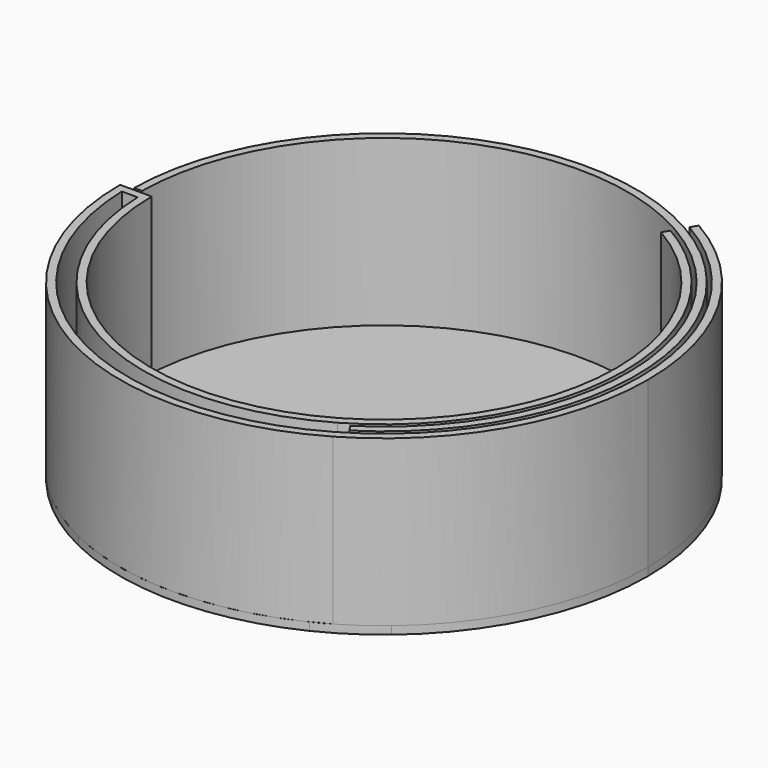
from build123d import *

# Parameters (mm, degrees)
F1_DEPTH = 1.2
F3_DEPTH = 25


with BuildPart() as f1:
    # F0 (on Top) → F1 (new body)
    with BuildSketch(Plane.XY):
        with BuildLine():
            ThreePointArc((25.666348, -30.679612), (36.239853, -16.931422), (40, 0))
            ThreePointArc((40, 0), (-16.931422, 36.239853), (-25.666348, -30.679612))
            ThreePointArc((-25.666348, -30.679612), (-21.736946, -33.578344), (-17.483625, -35.976699))
            ThreePointArc((-17.483625, -35.976699), (0, -40), (17.483625, -35.976699))
            ThreePointArc((17.483625, -35.976699), (21.736946, -33.578344), (25.666348, -30.679612))
        make_face()
    extrude(amount=F1_DEPTH)

    # F2 (on face) → F3 (join)
    with BuildSketch(Plane.XY.offset(1.2)):
        with BuildLine():
            ThreePointArc((20, -34.641016), (34.641016, -20), (40, 0))
            ThreePointArc((40, 0), (34.641016, 20), (20, 34.641016))
            Line((20, 34.641016), (19.4, 33.601786))
            ThreePointArc((19.4, 33.601786), (33.601786, 19.4), (38.8, 0))
            ThreePointArc((38.8, 0), (33.601786, -19.4), (19.4, -33.601786))
            Line((19.4, -33.601786), (20, -34.641016))
        make_face()
        with BuildLine():
            ThreePointArc((-40, 0), (-20, -34.641016), (20, -34.641016))
            Line((20, -34.641016), (19.4, -33.601786))
            ThreePointArc((19.4, -33.601786), (-18.878002, -33.897803), (-38.781439, -1.2))
            ThreePointArc((-38.781439, -1.2), (-38.795359, -0.600072), (-38.8, 0))
            Line((-38.8, 0), (-40, 0))
        make_face()
        with BuildLine():
            Line((18.5, 32.04294), (19.1, 33.08217))
            ThreePointArc((19.1, 33.08217), (-18.920896, 33.184932), (-38.197768, 0.412973))
            Line((-38.197768, 0.412973), (-36.997838, 0.4))
            ThreePointArc((-36.997838, 0.4), (-18.326522, 32.142473), (18.5, 32.04294))
        make_face()
        with BuildLine():
            ThreePointArc((20.512714, -32.225279), (38.191066, 0.826139), (19.1, 33.08217))
            Line((19.1, 33.08217), (18.5, 32.04294))
            ThreePointArc((18.5, 32.04294), (36.991346, 0.800187), (19.868335, -31.212966))
            Line((19.868335, -31.212966), (20.512714, -32.225279))
        make_face()
        with BuildLine():
            Line((17.6, -30.484094), (18.2, -31.523325))
            ThreePointArc((18.2, -31.523325), (31.523325, -18.2), (36.4, 0))
            ThreePointArc((36.4, 0), (31.523325, 18.2), (18.2, 31.523325))
            Line((18.2, 31.523325), (17.6, 30.484094))
            ThreePointArc((17.6, 30.484094), (30.484094, 17.6), (35.2, 0))
            ThreePointArc((35.2, 0), (30.484094, -17.6), (17.6, -30.484094))
        make_face()
        with BuildLine():
            ThreePointArc((-36.380214, -1.2), (-17.677841, -31.819081), (18.2, -31.523325))
            Line((18.2, -31.523325), (17.6, -30.484094))
            ThreePointArc((17.6, -30.484094), (-17.6, -30.484094), (-35.2, 0))
            Line((-35.2, 0), (-36.4, 0))
            ThreePointArc((-36.4, 0), (-36.395053, -0.600082), (-36.380214, -1.2))
        make_face()
        with BuildLine():
            Line((-36.4, 0), (-38.8, 0))
            ThreePointArc((-38.8, 0), (-38.795359, -0.600072), (-38.781439, -1.2))
            Line((-38.781439, -1.2), (-36.380214, -1.2))
            ThreePointArc((-36.380214, -1.2), (-36.395053, -0.600082), (-36.4, 0))
        make_face()
    extrude(amount=F3_DEPTH)


solid = f1.part
